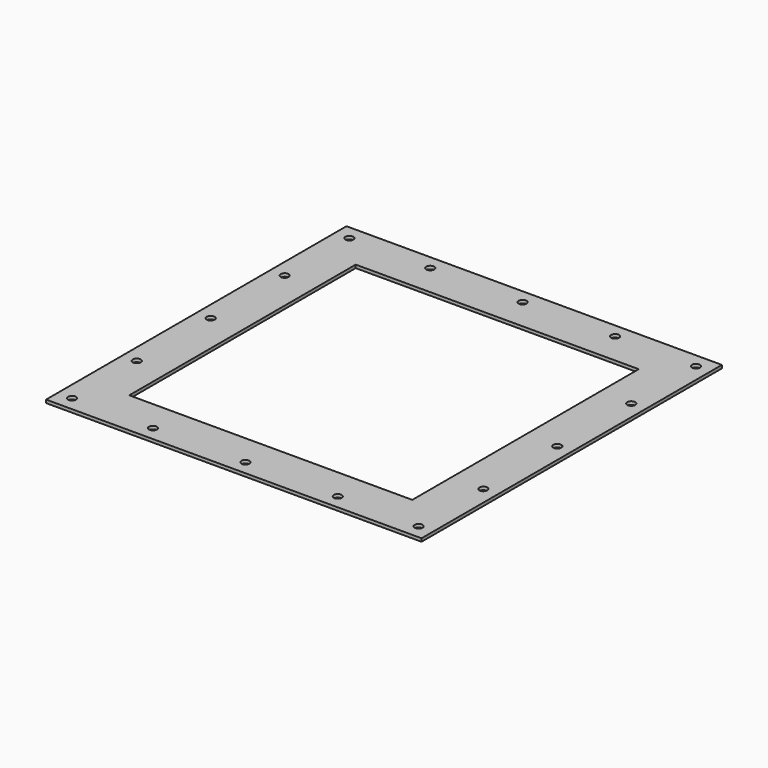
from build123d import *

# Parameters (mm, degrees)
F0_W            = 412.75
F0_H            = 412.75
F0_W_2          = 311.15
F0_H_2          = 311.15
F1_DEPTH        = 3.429
F2_D            = 8.7376
F2_COPIES_COUNT = 4


# Not quite as in the source:
# - a pattern or mirror of a feature is missing from the dataset's text; its kind, count and spacing are read off the source's solid


with BuildPart() as f1:
    # F0 (on Top) → F1 (new body)
    with BuildSketch(Plane.XY):
        Rectangle(F0_W, F0_H)
        Rectangle(F0_W_2, F0_H_2, mode=Mode.SUBTRACT)
    extrude(amount=-F1_DEPTH)

    # F2 (through all)
    with Locations(Plane.XY):
        with Locations((-190.5, 190.5), (-101.6, 190.5), (0, 190.5), (101.6, 190.5), (190.5, 190.5)):
            f2 = Hole(F2_D / 2)

    # F2_copies: F2 ×4 about axis
    f2_copies_axis = Axis((0, 0, 0), (0, 0, 1))
    for i in range(1, F2_COPIES_COUNT):
        add(f2.rotate(f2_copies_axis, i * 360 / F2_COPIES_COUNT), mode=Mode.SUBTRACT)


solid = f1.part
